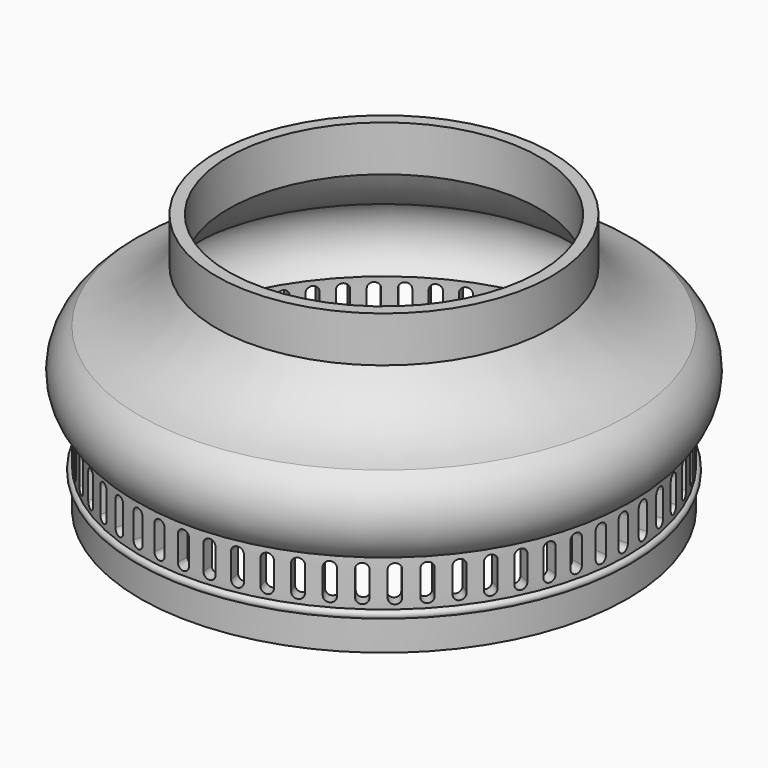
from build123d import *

# Parameters (mm, degrees)
F4_DEPTH        = 2540
F4_COPIES_COUNT = 60
F5_W            = 8.6182653904
F5_H            = 4.8653250911
F6_DEPTH        = 2540


# Not quite as in the source:
# - a pattern or mirror of a feature is missing from the dataset's text; its kind, count and spacing are read off the source's solid


with BuildPart() as f2:
    # F0 (on Front) → F2 (revolve)
    with BuildSketch(Plane.XZ):
        with BuildLine():
            Line((96.6, -107.95), (101.6, -107.95))
            Line((101.6, -107.95), (101.6, -95.25))
            ThreePointArc((101.6, -95.25), (103.1875, -93.6625), (101.6, -92.075))
            Line((101.6, -92.075), (101.6, -73.025))
            ThreePointArc((101.6, -73.025), (109.9683697671, -56.9892826945), (101.6, -40.9535653889))
            ThreePointArc((101.6, -40.9535653889), (83.3860437577, -33.3921832697), (69.85, -19.05))
            Line((69.85, -19.05), (69.85, 0))
            Line((69.85, 0), (64.85, 0))
            Line((64.85, 0), (64.85, -19.05))
            ThreePointArc((64.85, -19.05), (77.7823135338, -35.6042725114), (96.6, -44.9414748641))
            ThreePointArc((96.6, -44.9414748641), (103.3617914925, -58.983237432), (96.6, -73.025))
            Line((96.6, -73.025), (96.6, -107.95))
        make_face()
    revolve(axis=Axis((0, 0, -37.3326065019), (0, 0, -1)))

    # F3 (on Right) → F4 (cut)
    with BuildSketch(Plane.YZ):
        Polygon((-0.0027141112, -87.6582702), (0.0082051842, -77.4417296052), (-4.7271141112, -77.4417296052), (-4.7271141112, -87.8855058875), align=None)
        with BuildLine():
            Line((-4.7271141112, -77.4417296052), (0.0082051842, -77.4417296052))
            ThreePointArc((0.0082051842, -77.4417296052), (-2.3594544635, -75.0715380837), (-4.7271141112, -77.4417296052))
        make_face()
        with BuildLine():
            ThreePointArc((-4.7271141112, -87.8855058875), (-2.2457000919, -90.2504367225), (-0.0027141112, -87.6582702))
            Line((-0.0027141112, -87.6582702), (-4.7271141112, -87.8855058875))
        make_face()
    f4 = extrude(amount=F4_DEPTH, mode=Mode.SUBTRACT)

    # F4_copies: F4 ×60 about axis
    f4_copies_axis = Axis((0, 0, 0), (0, 0, 1))
    for i in range(1, F4_COPIES_COUNT):
        add(f4.rotate(f4_copies_axis, i * 360 / F4_COPIES_COUNT), mode=Mode.SUBTRACT)

    # F5 (on Right) → F6 (cut)
    with BuildSketch(Plane.YZ):
        with Locations((37.7049073577, -101.6000029456)):
            Rectangle(F5_W, F5_H)
        with BuildLine():
            ThreePointArc((42.0140400529, -104.0326654911), (44.4467025984, -101.6000029456), (42.0140400529, -99.1673404))
            Line((42.0140400529, -99.1673404), (42.0140400529, -104.0326654911))
        make_face()
        with BuildLine():
            Line((33.3957746625, -104.0326654911), (33.3957746625, -99.1673404))
            ThreePointArc((33.3957746625, -99.1673404), (30.9631121169, -101.6000029456), (33.3957746625, -104.0326654911))
        make_face()
        Polygon((9.3502895907, -99.1673404), (-1.9651199691, -99.1673404), (-3.8829869591, -99.1673404), (-3.8829869591, -107.95), (0, -107.9670339823), (0, -104.0326654911), (9.3502895907, -104.0326654911), (9.3502895907, -103.3471207142), align=None)
    extrude(amount=-F6_DEPTH, mode=Mode.SUBTRACT)


solid = f2.part
